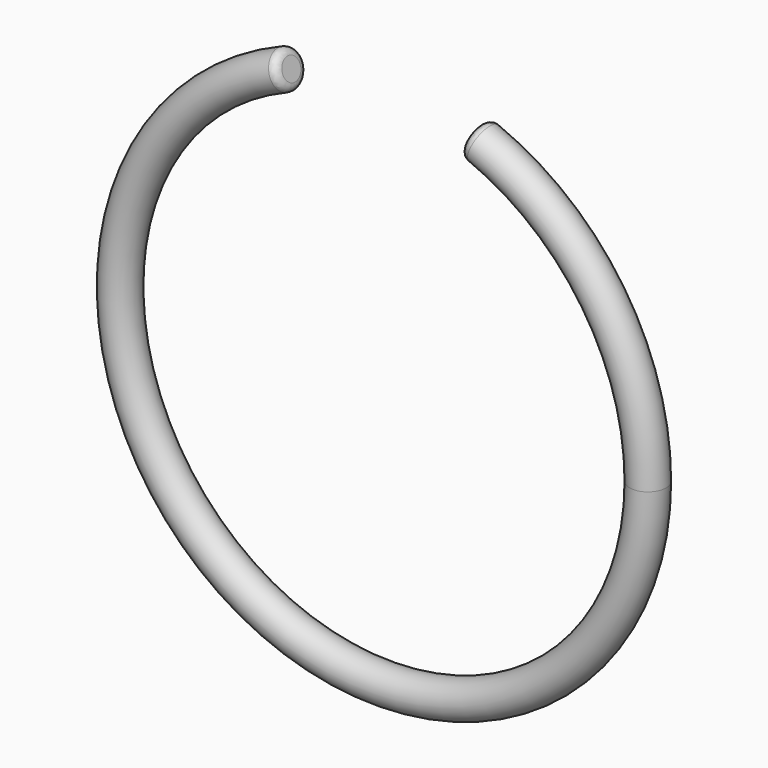
from build123d import *

# Parameters (mm, degrees)
F1_R     = 0.5
F4_DEPTH = 12.5
F5_R     = 0.2


with BuildPart() as f2:
    # F2: sweep along a path in F0
    with BuildLine(Plane.XZ) as f2_path:
        CenterArc((0, 0), 7.25, 0, 360)
    # F1 (on Top) → F2 (sweep)
    with BuildSketch(Plane.XY):
        with Locations((7.25, 0)):
            Circle(F1_R)
    sweep(path=f2_path.line)

    # F3 (on Front) → F4 (cut, symmetric)
    with BuildSketch(Plane.XZ):
        Polygon((-3, 8), (0, 0), (3, 8), align=None)
    extrude(amount=F4_DEPTH, both=True, mode=Mode.SUBTRACT)

    # F5
    f5_edges = [f2.edges().sort_by_distance(p)[0] for p in [
        (-2.370083, 0, 6.320222),
        (2.370083, 0, 6.320222),
    ]]
    fillet(f5_edges, radius=F5_R)


solid = f2.part
